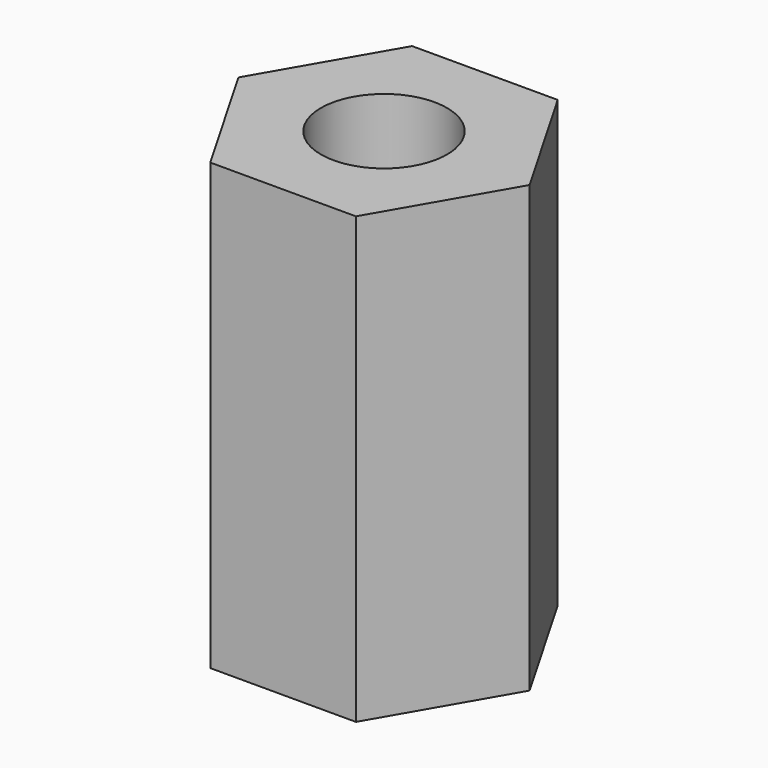
from build123d import *

# Parameters (mm, degrees)
F1_DEPTH = 30
F3_D     = 8.5


with BuildPart() as f1:
    # F0 (on Top) → F1 (new body)
    with BuildSketch(Plane.XY):
        Polygon((4.9074772881, 8.5), (-4.9074772881, 8.5), (-9.8149545762, 0), (-4.9074772881, -8.5), (4.9074772881, -8.5), (9.8149545762, 0), align=None)
    extrude(amount=F1_DEPTH)

    # F3 (through all)
    with Locations(Plane.XY.offset(30)):
        with Locations((0, 0)):
            Hole(F3_D / 2)


solid = f1.part
